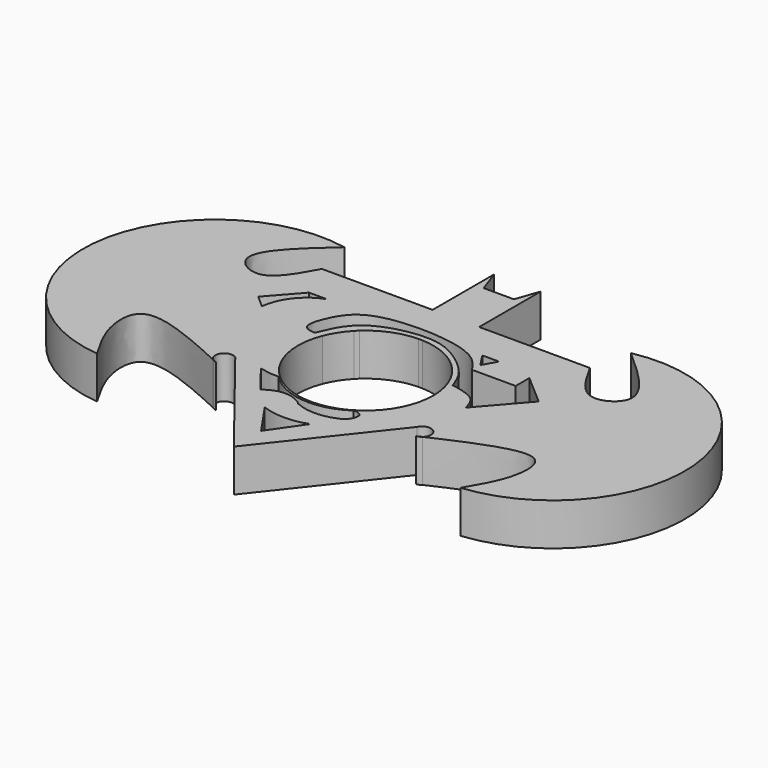
from build123d import *

# Parameters (mm, degrees)
F1_DEPTH = 7


# Not quite as in the source:
# - a feature names something its author has since deleted; it is built from what else it names


with BuildPart() as f1:
    # F0 (on Top) → F1 (new body)
    with BuildSketch(Plane.XY):
        with BuildLine():
            ThreePointArc((16.5792349726, -10.2448631078), (16.9834682398, -10.1267607204), (17.3376568133, -9.8989380643))
            add(Edge.make_bspline(
                [(17.3376568133, -9.8989380643), (17.0850021821, -10.01408297), (16.8321185773, -10.1294730389), (16.5792349726, -10.2448631078)],
                knots=[0.9832167043, 0.9832167043, 0.9832167043, 0.9832167043, 1, 1, 1, 1], degree=3))
        make_face()
    extrude(amount=F1_DEPTH)


with BuildPart() as f1b:
    # F0 (on Top) → F1, piece 2 (new body)
    with BuildSketch(Plane.XY):
        with BuildLine():
            add(Edge.make_bspline(
                [(-17.3376568133, -9.8989380643), (-17.0850021821, -10.01408297), (-16.8321185773, -10.1294730389), (-16.5792349726, -10.2448631078)],
                knots=[0.9832167043, 0.9832167043, 0.9832167043, 0.9832167043, 1, 1, 1, 1], degree=3))
            ThreePointArc((-17.3376568133, -9.8989380643), (-16.9834682398, -10.1267607204), (-16.5792349726, -10.2448631078))
        make_face()
    extrude(amount=F1_DEPTH)


with BuildPart() as f1c:
    # F0 (on Top) → F1, piece 3 (new body)
    with BuildSketch(Plane.XY):
        with BuildLine():
            Line((-3.8506640121, 25.8194226772), (-3.8506640121, 18.6837073416))
            Line((-3.8506640121, 18.6837073416), (-22.1720933914, 18.6837073416))
            add(Edge.make_bspline(
                [(-22.1720933914, 18.6837073416), (-23.7664845821, 15.772799918), (-26.5823710911, 10.6317874798), (-34.6816663683, 15.4985414684), (-27.9134744848, 21.511081938), (-23.7149503082, 25.2408515662)],
                knots=[0, 0, 0, 0, 0.3313598243, 0.5852212834, 1, 1, 1, 1], degree=3))
            ThreePointArc((-23.7149503082, 25.2408515662), (-49.5692789527, 6.9809498228), (-30.0792362541, -17.9591495544))
            add(Edge.make_bspline(
                [(-30.0792362541, -17.9591495544), (-31.4287635496, -15.6693361188), (-33.8865169415, -11.4991375929), (-33.716724634, -2.5786683332), (-23.7541469989, -6.9746846915), (-17.3376568133, -9.8989380643)],
                knots=[0, 0, 0, 0, 0.3058338248, 0.5569832657, 0.9832167043, 0.9832167043, 0.9832167043, 0.9832167043], degree=3))
            ThreePointArc((-17.3376568133, -9.8989380643), (-17.2546789352, -7.6115300309), (-15.0363789871, -8.1756808795))
            Line((-15.0363789871, -8.1756808795), (0, -27.2537693381))
            Line((0, -27.2537693381), (15.0363789871, -8.1756808795))
            ThreePointArc((15.0363789871, -8.1756808795), (17.2546789352, -7.6115300309), (17.3376568133, -9.8989380643))
            add(Edge.make_bspline(
                [(30.0792362541, -17.9591495544), (31.4287635496, -15.6693361188), (33.8865169415, -11.4991375929), (33.716724634, -2.5786683332), (23.7541469989, -6.9746846915), (17.3376568133, -9.8989380643)],
                knots=[0, 0, 0, 0, 0.3058338248, 0.5569832657, 0.9832167043, 0.9832167043, 0.9832167043, 0.9832167043], degree=3))
            ThreePointArc((30.0792362541, -17.9591495544), (49.5692789527, 6.9809498228), (23.7149503082, 25.2408515662))
            add(Edge.make_bspline(
                [(22.1720933914, 18.6837073416), (23.7664845821, 15.772799918), (26.5823710911, 10.6317874798), (34.6816663683, 15.4985414684), (27.9134744848, 21.511081938), (23.7149503082, 25.2408515662)],
                knots=[0, 0, 0, 0, 0.3313598243, 0.5852212834, 1, 1, 1, 1], degree=3))
            Line((22.1720933914, 18.6837073416), (3.8506640121, 18.6837073416))
            Line((3.8506640121, 18.6837073416), (3.8506640121, 25.8194226772))
            Line((3.8506640121, 25.8194226772), (3.8506640121, 31.412281096))
            Line((3.8506640121, 31.412281096), (2.5006639771, 27.5551360101))
            Line((2.5006639771, 27.5551360101), (0, 27.5551360101))
            Line((0, 27.5551360101), (-2.5006639771, 27.5551360101))
            Line((-2.5006639771, 27.5551360101), (-3.8506640121, 31.412281096))
            Line((-3.8506640121, 31.412281096), (-3.8506640121, 25.8194226772))
        make_face()
        Polygon((-20.2526636422, 15.1130193844), (0, 15.1130193844), (20.2526636422, 15.1130193844), (26.1378940195, 8.3870412782), (0, -24.7384030372), (-26.1378940195, 8.3870412782), align=None, mode=Mode.SUBTRACT)
        Polygon((20.2526636422, 15.1130193844), (0, 15.1130193844), (-20.2526636422, 15.1130193844), (-26.1378940195, 8.3870412782), (0, -24.7384030372), (26.1378940195, 8.3870412782), align=None)
        with BuildLine():
            Line((0, -21.6201487929), (-3.766995389, -16.1573626101))
            ThreePointArc((-3.766995389, -16.1573626101), (0, -16.8352683554), (3.766995389, -16.1573626101))
            Line((3.766995389, -16.1573626101), (0, -21.6201487929))
        make_face(mode=Mode.SUBTRACT)
        with BuildLine():
            add(Edge.make_bspline(
                [(11.3654661838, 3.8127656249), (11.0702905387, 3.8658966707), (10.7717963194, 3.9170817546), (10.4734106347, 3.9683333625)],
                knots=[0.9102418538, 0.9102418538, 0.9102418538, 0.9102418538, 1, 1, 1, 1], degree=3))
            ThreePointArc((10.4734106347, 3.9683333625), (10.5184572741, -3.8473440933), (5.4412195451, -9.7894397114))
            ThreePointArc((5.4412195451, -9.7894397114), (5.6124095819, -9.7340283467), (5.7888518665, -9.6987499078))
            ThreePointArc((5.7888518665, -9.6987499078), (6.5915164137, -9.7983213926), (7.2357721967, -10.2873196974))
            ThreePointArc((7.2357721967, -10.2873196974), (6.8639840342, -11.7423461015), (5.6799273007, -12.666109018))
            ThreePointArc((5.6799273007, -12.666109018), (2.3573584338, -13.3979774494), (-0.9739922243, -12.7071822062))
            ThreePointArc((-0.9739922243, -12.7071822062), (-4.1081974234, -11.4743163831), (-7.2582499124, -12.666109018))
            Line((-7.2582499124, -12.666109018), (-9.4156803641, -9.9287711898))
            Line((-9.4156803641, -9.9287711898), (-10.9763270325, -7.9509104535))
            add(Edge.make_bspline(
                [(-10.9763270325, -7.9509104535), (-10.3428475671, -8.1020396785), (-9.2143948724, -8.3670340298), (-8.1833899777, -8.3551484222), (-7.7320225253, -8.3383332333)],
                knots=[0, 0, 0, 0, 0.5203503372, 0.9269013897, 0.9269013897, 0.9269013897, 0.9269013897], degree=3))
            add(Edge.make_bspline(
                [(-7.7320225253, -8.3383332333), (-7.6508658457, -8.3353098321), (-7.569736476, -8.3319113533), (-7.488530354, -8.3283799827)],
                knots=[0.9269013897, 0.9269013897, 0.9269013897, 0.9269013897, 1, 1, 1, 1], degree=3))
            ThreePointArc((-7.488530354, -8.3283799827), (-10.9005534004, -2.572534852), (-10.421984849, 4.1014914125))
            add(Edge.make_bspline(
                [(-11.7478008935, 4.1423421903), (-11.3286185316, 4.111655498), (-10.8755128269, 4.1066551355), (-10.421984849, 4.1014914125)],
                knots=[0.9507604249, 0.9507604249, 0.9507604249, 0.9507604249, 1, 1, 1, 1], degree=3))
            add(Edge.make_bspline(
                [(10.6188114733, 8.7546054274), (9.7238694578, 10.0752930999), (7.317364425, 13.6266079113), (-9.4942346395, 14.2413402565), (-13.0198623921, 8.8144018215), (-14.3381284396, 4.6074785308), (-12.5637633708, 4.2020755945), (-11.7478008935, 4.1423421903)],
                knots=[0, 0, 0, 0, 0.1869763466, 0.5029361243, 0.7033603953, 0.8549127717, 0.9507604249, 0.9507604249, 0.9507604249, 0.9507604249], degree=3))
            Line((10.6188114733, 8.7546054274), (12.9112154245, 8.7546054274))
            Line((12.9112154245, 8.7546054274), (14.2252305523, 8.7546054274))
            Line((14.2252305523, 8.7546054274), (17.8316496313, 8.7546054274))
            Line((17.8316496313, 8.7546054274), (17.8316496313, 11.5920095704))
            Line((17.8316496313, 11.5920095704), (22.8700302541, 7.2163445875))
            Line((22.8700302541, 7.2163445875), (16.6028764442, 0))
            add(Edge.make_bspline(
                [(16.6028764442, 0), (16.3378800898, 0.9165232113), (15.7718233446, 2.8802807514), (12.9602593254, 3.5257059408), (11.3654661838, 3.8127656249)],
                knots=[0, 0, 0, 0, 0.4252910171, 0.9102418538, 0.9102418538, 0.9102418538, 0.9102418538], degree=3))
        make_face(mode=Mode.SUBTRACT)
        with BuildLine():
            Line((-21.6983128122, 5.6717018071), (-23.7482488155, 7.4817519635))
            Line((-23.7482488155, 7.4817519635), (-19.3462949246, 12.4670965597))
            Line((-19.3462949246, 12.4670965597), (-16.4293367416, 12.4670965597))
            ThreePointArc((-16.4293367416, 12.4670965597), (-20.0285535224, 9.8174252893), (-21.6983128122, 5.6717018071))
        make_face(mode=Mode.SUBTRACT)
        Polygon((10.6188114733, 10.4517443106), (9.1338139027, 12.7322748303), (11.8916649371, 12.7322748303), align=None, mode=Mode.SUBTRACT)
        with BuildLine():
            ThreePointArc((5.7888518665, -9.6987499078), (5.6124095819, -9.7340283467), (5.4412195451, -9.7894397114))
            ThreePointArc((5.4412195451, -9.7894397114), (5.2779102429, -9.878444385), (5.1131454862, -9.9647249454))
            ThreePointArc((5.1131454862, -9.9647249454), (4.8515858311, -10.0946577417), (4.5867272221, -10.2177264296))
            ThreePointArc((4.5867272221, -10.2177264296), (4.2266476764, -10.3718585326), (3.8613989114, -10.5133057811))
            ThreePointArc((3.8613989114, -10.5133057811), (0.9071691587, -11.1632004424), (-2.1132312692, -10.998829647))
            ThreePointArc((-2.1132312692, -10.998829647), (-2.4633866315, -10.9257368769), (-2.8110292899, -10.8414996348))
            ThreePointArc((-2.8110292899, -10.8414996348), (-5.3008654775, -9.8661454069), (-7.488530354, -8.3283799827))
            add(Edge.make_bspline(
                [(-7.7320225253, -8.3383332333), (-7.6508658457, -8.3353098321), (-7.569736476, -8.3319113533), (-7.488530354, -8.3283799827)],
                knots=[0.9269013897, 0.9269013897, 0.9269013897, 0.9269013897, 1, 1, 1, 1], degree=3))
            ThreePointArc((-7.7320225253, -8.3383332333), (-1.22270189, -11.5143324097), (5.7888518665, -9.6987499078))
        make_face()
        with BuildLine():
            ThreePointArc((-7.5748789973, 8.2499217073), (-4.1434483054, 10.4053753484), (-0.1696203788, 11.1987155034))
            Line((-0.1696203788, 11.1987155034), (0.4601464831, 11.190543562))
            ThreePointArc((0.4601464831, 11.190543562), (6.551774405, 9.0837355832), (10.4734106347, 3.9683333625))
            add(Edge.make_bspline(
                [(11.3654661838, 3.8127656249), (11.0702905387, 3.8658966707), (10.7717963194, 3.9170817546), (10.4734106347, 3.9683333625)],
                knots=[0.9102418538, 0.9102418538, 0.9102418538, 0.9102418538, 1, 1, 1, 1], degree=3))
            add(Edge.make_bspline(
                [(-11.7478008927, 4.1423421862), (-11.1941041625, 5.4902929916), (-10.0555326267, 8.2507614708), (-6.2924585186, 11.3146577634), (1.4560057353, 12.7730545434), (6.2091952943, 10.5462199473), (10.0831340079, 7.2322332261), (10.961497048, 4.890959233), (11.3654661838, 3.8127656249)],
                knots=[0.0009795765, 0.0009795765, 0.0009795765, 0.0009795765, 0.1555024095, 0.3177552589, 0.5229639524, 0.6937681454, 0.8590519191, 1, 1, 1, 1], degree=3))
            add(Edge.make_bspline(
                [(-11.7478008935, 4.1423421903), (-11.3286185316, 4.111655498), (-10.8755128269, 4.1066551355), (-10.421984849, 4.1014914125)],
                knots=[0.9507604249, 0.9507604249, 0.9507604249, 0.9507604249, 1, 1, 1, 1], degree=3))
            ThreePointArc((-10.421984849, 4.1014914125), (-9.4341404452, 6.0363063259), (-8.0913616782, 7.7440213193))
            ThreePointArc((-8.0913616782, 7.7440213193), (-7.837203457, 8.0011400421), (-7.5748789973, 8.2499217073))
        make_face()
    extrude(amount=F1_DEPTH)


solid = Compound([f1.part, f1b.part, f1c.part])
